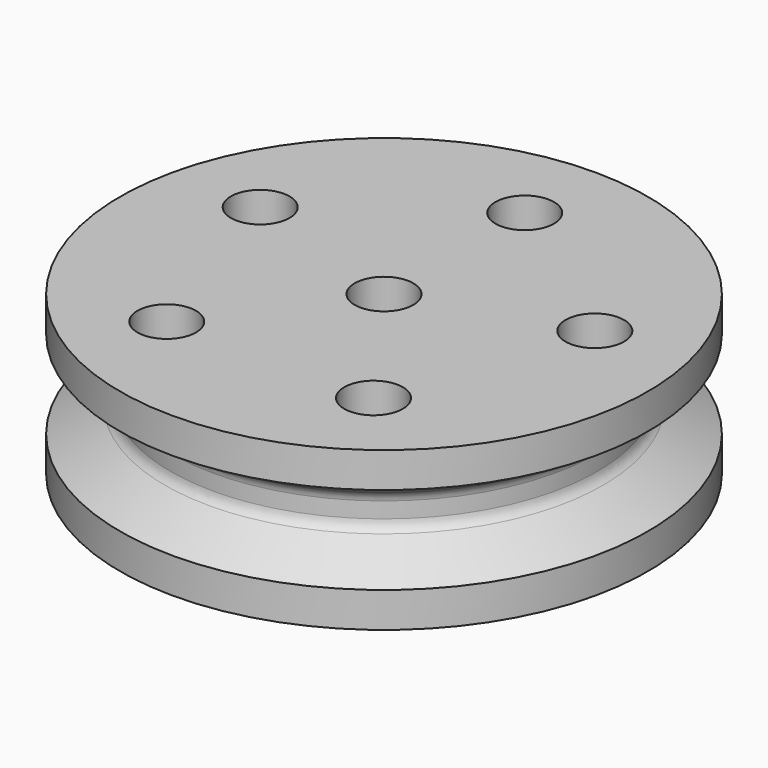
from build123d import *

# Parameters (mm, degrees)
F2_R     = 5
F3_DEPTH = 27
F4_R     = 2


# Not quite as in the source:
# - a feature names something its author has since deleted; it is built from what else it names


with BuildPart() as f1:
    # F0 (on Right) → F1 (revolve)
    with BuildSketch(Plane.YZ):
        Polygon((-5, -11), (-5, 16), (-45, 16), (-45, 10), (-36.3397459622, 5), (-36.3397459622, 0), (-45, -5), (-45, -11), align=None)
    revolve(axis=Axis((0, 0, -0.4931497392), (0, 0, -1)))

    # F2 (on face) → F3 (cut, through all)
    with BuildSketch(Plane.XY.offset(16)):
        with Locations((-28.5316954889, 9.2705098312)):
            Circle(F2_R)
        with Locations((-17.6335575688, -24.2705098312)):
            Circle(F2_R)
        with Locations((17.6335575688, -24.2705098312)):
            Circle(F2_R)
        with Locations((28.5316954889, 9.2705098312)):
            Circle(F2_R)
        with Locations((0, 30)):
            Circle(F2_R)
    extrude(amount=-F3_DEPTH, mode=Mode.SUBTRACT)

    # F4
    f4_edges = [f1.edges().sort_by_distance(p)[0] for p in [
        (0, 36.339746, 0),
        (0, 36.339746, 5),
    ]]
    fillet(f4_edges, radius=F4_R)


solid = f1.part
